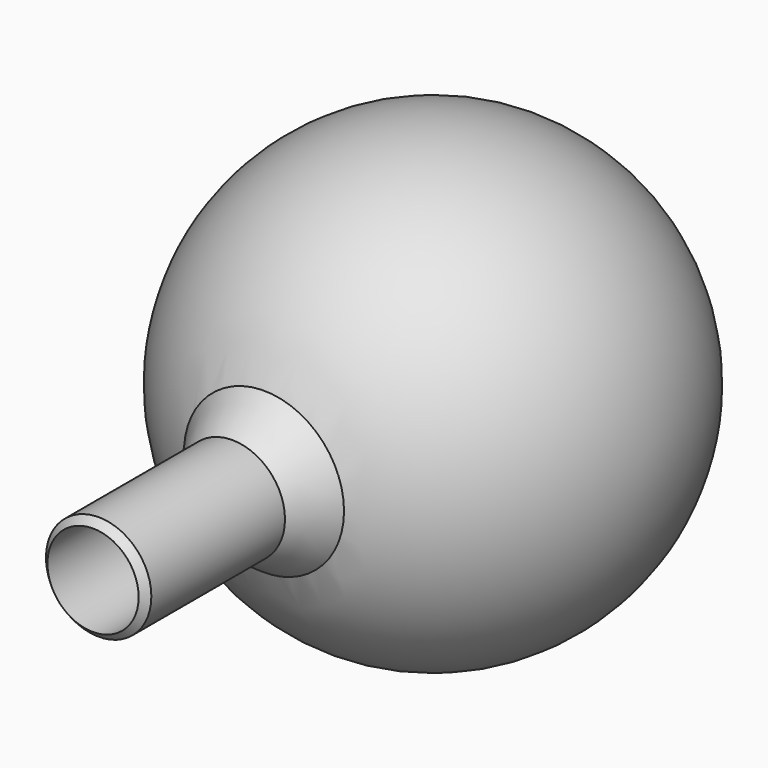
from build123d import *

# Parameters (mm, degrees)
F2_R     = 18.6597493024
F3_DEPTH = 163
F4_T     = -2.5


# Not quite as in the source:
# - a fillet or chamfer that OpenCascade refuses, or shapes differently, is made with other operations: its cross-section is extruded or revolved along the edge and cut away or added


with BuildPart() as f1:
    # F0 (on Top) → F1 (revolve)
    with BuildSketch(Plane.XY):
        with BuildLine():
            Line((-80, 0), (80, 0))
            ThreePointArc((80, 0), (0, 80), (-80, 0))
        make_face()
    revolve(axis=Axis((0, 0, 0), (-1, 0, 0)))

    # F2 (on Front) → F3 (join)
    with BuildSketch(Plane.XZ):
        Circle(F2_R)
    extrude(amount=F3_DEPTH)

    # F4
    f4_openings = [f1.faces().sort_by_distance(p)[0] for p in [
        (0, -163, 0),
    ]]
    offset(amount=F4_T, openings=f4_openings, kind=Kind.INTERSECTION)

    # F5: chamfer of 15 on 3 edges, made by hand

    # F5_s1 → F5_t2 (revolve)
    with BuildSketch(Plane.XY):
        with BuildLine():
            Line((28.3450520489, -74.8101465352), (18.6597493072, -88.8370490105))
            Line((18.6597493072, -88.8370490105), (18.6597493024, -77.7934043218))
            ThreePointArc((18.6597493024, -77.7934043218), (23.7757008768, -76.3853130389), (28.3450520489, -74.8101465352))
        make_face()
    revolve(axis=Axis((2.4e-09, -77.7934043218, -1e-10), (0, -1, 0)))

    # F5_s3 → F5_t4 (revolve, cut)
    with BuildSketch(Plane.XY):
        Polygon((18.6597493024, -148), (3.6597493024, -163), (18.6597493024, -163), align=None)
    revolve(axis=Axis((0, -163, 0), (0, -1, 0)), mode=Mode.SUBTRACT)


solid = f1.part
